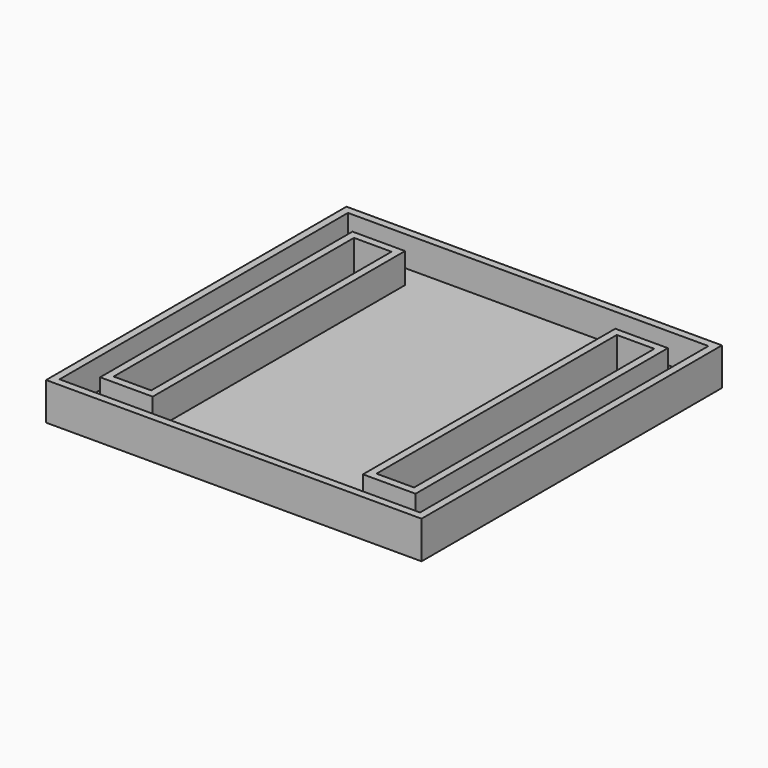
from build123d import *

# Parameters (mm, degrees)
F0_W     = 127
F0_H     = 127
F0_W_2   = 12.7
F0_H_2   = 101.6
F1_DEPTH = 12.7
F2_T     = -2.54


with BuildPart() as f1:
    # F0 (on Top) → F1 (new body)
    with BuildSketch(Plane.XY):
        with Locations((13.4799859107, -4.1653172493)):
            Rectangle(F0_W, F0_H)
        with Locations((-30.9700140893, -4.1653172493)):
            Rectangle(F0_W_2, F0_H_2, mode=Mode.SUBTRACT)
        with Locations((57.9299859107, -4.1653172493)):
            Rectangle(F0_W_2, F0_H_2, mode=Mode.SUBTRACT)
    extrude(amount=F1_DEPTH)

    # F2
    f2_openings = [f1.faces().sort_by_distance(p)[0] for p in [
        (13.479986, -4.165317, 12.7),
    ]]
    offset(amount=F2_T, openings=f2_openings, kind=Kind.INTERSECTION)


solid = f1.part
